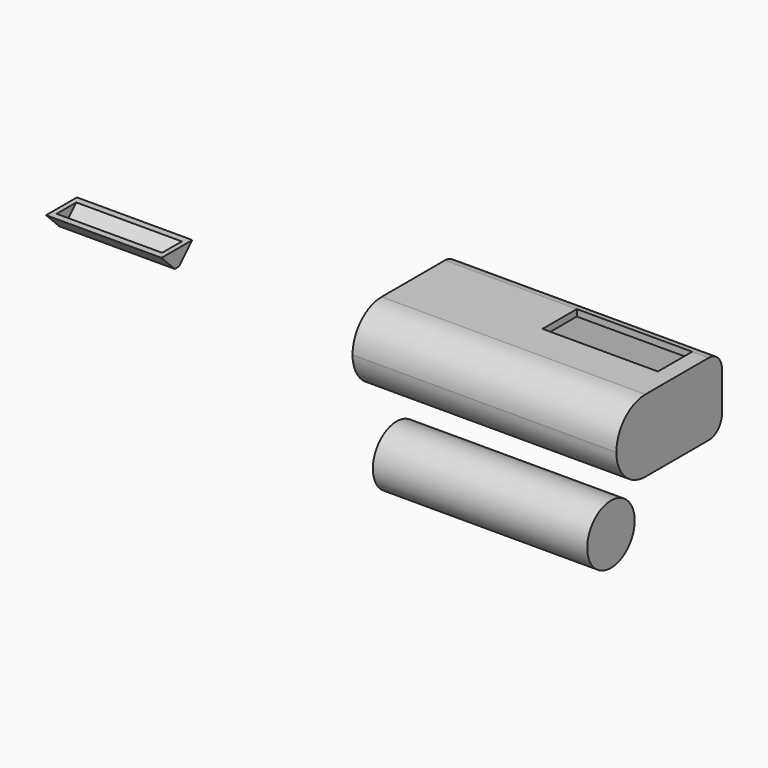
from build123d import *

# Parameters (mm, degrees)
F0_W        = 80
F0_H        = 40
F1_DEPTH    = 22
F2_R        = 10.99999
F3_W        = 35
F3_H        = 13
F4_DEPTH    = 2
F5_R        = 4.99999
F6_W        = 35
F6_H        = 11.8533317
F7_DEPTH    = 5
F8_T1_DEPTH = 61.1282991577
F9_T        = -1.5
F10_W       = 32
F10_H       = 1.6933317
F11_DEPTH   = 2
F12_R       = 9
F13_DEPTH   = 65
F14_R       = 9
F15_DEPTH   = 78
F16_W       = 16
F16_H       = 18
F17_DEPTH   = 78


# Not quite as in the source:
# - a fillet or chamfer that OpenCascade refuses, or shapes differently, is made with other operations: its cross-section is extruded or revolved along the edge and cut away or added
# - a fillet or chamfer is up to 0.001 mm smaller than in the source, because OpenCascade refuses the exact size


with BuildPart() as f1:
    # F0 (on Top) → F1 (new body)
    with BuildSketch(Plane.XY):
        Rectangle(F0_W, F0_H)
    extrude(amount=F1_DEPTH)

    # F2 (radius 11 in the source; OpenCascade refuses exactly that, so slightly less here)
    f2_edges = [f1.edges().sort_by_distance(p)[0] for p in [
        (0, -20, 22),
        (0, -20, 0),
    ]]
    fillet(f2_edges, radius=F2_R)

    # F3 (on face) → F4 (cut)
    with BuildSketch(Plane.XY.offset(22)):
        with Locations((17.5, 8.5)):
            Rectangle(F3_W, F3_H)
    extrude(amount=-F4_DEPTH, mode=Mode.SUBTRACT)

    # F5 (radius 5 in the source; OpenCascade refuses exactly that, so slightly less here)
    f5_edges = [f1.edges().sort_by_distance(p)[0] for p in [
        (0, 20, 22),
        (0, 20, 0),
    ]]
    fillet(f5_edges, radius=F5_R)

    # F14 (on face) → F15 (cut)
    with BuildSketch(Plane(origin=(-40, 0, 0), x_dir=(0, -1, 0), z_dir=(-1, 0, 0))):
        with Locations((9, 11)):
            Circle(F14_R)
    extrude(amount=-F15_DEPTH, mode=Mode.SUBTRACT)

    # F16 (on face) → F17 (cut)
    with BuildSketch(Plane(origin=(-40, 0, 0), x_dir=(0, -1, 0), z_dir=(-1, 0, 0))):
        with Locations((-10, 11)):
            Rectangle(F16_W, F16_H)
    extrude(amount=-F17_DEPTH, mode=Mode.SUBTRACT)


with BuildPart() as f7:
    # F6 (on Top) → F7 (new body)
    with BuildSketch(Plane.XY):
        with Locations((-131.0947090387, 5.4316394962)):
            Rectangle(F6_W, F6_H)
    extrude(amount=F7_DEPTH)

    # F8: chamfer of 5.08 on 2 edges, made by hand

    # F8_s2 → F8_t1 (cut)
    with BuildSketch(Plane.YZ.offset(-161.6588586176)):
        Polygon((-0.4950263537, 5.08), (4.5849736463, 0), (-0.4950263537, 0), align=None)
        Polygon((11.3583053462, 5.08), (6.2783053462, 0), (11.3583053462, 0), align=None)
    extrude(amount=F8_T1_DEPTH, mode=Mode.SUBTRACT)

    # F9
    f9_openings = [f7.faces().sort_by_distance(p)[0] for p in [
        (-131.094709, 5.431639, 5),
    ]]
    offset(amount=F9_T, openings=f9_openings, kind=Kind.INTERSECTION)

    # F10 (on face) → F11 (cut)
    with BuildSketch(Plane(origin=(0, 0, 0), x_dir=(1, 0, 0), z_dir=(0, 0, -1))):
        with Locations((-131.0947090387, -5.4316394962)):
            Rectangle(F10_W, F10_H)
    extrude(amount=-F11_DEPTH, mode=Mode.SUBTRACT)


with BuildPart() as f13:
    # F12 (on Right) → F13 (new body)
    with BuildSketch(Plane.YZ):
        with Locations((-53.3060245216, 10.8038987964)):
            Circle(F12_R)
    extrude(amount=F13_DEPTH)


solid = Compound([f1.part, f7.part, f13.part])
